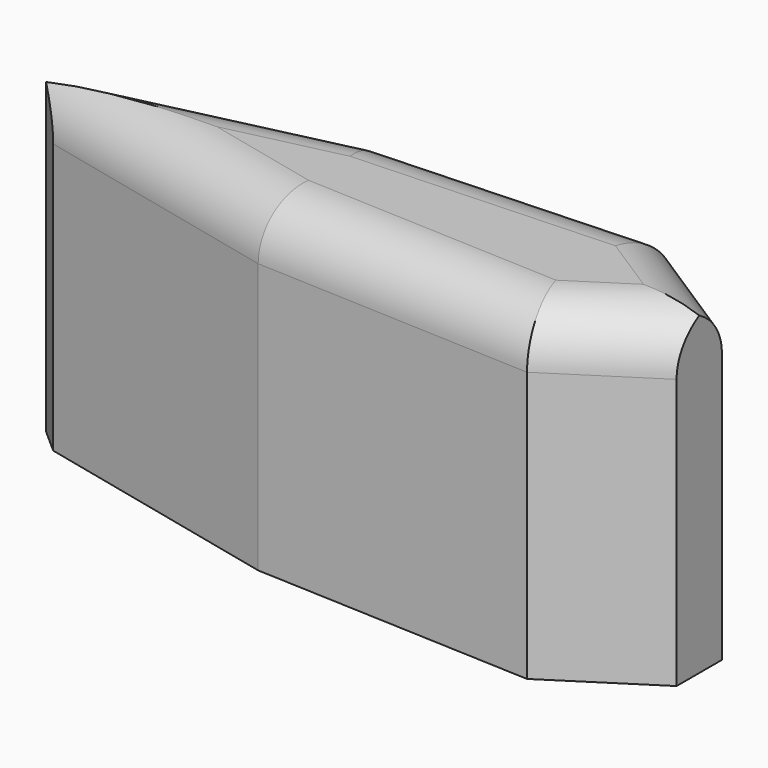
from build123d import *

# Parameters (mm, degrees)
F1_DEPTH     = 30
F2_T1_DEPTH  = 75.8181276712
F2_T3_DEPTH  = 75.8181276712
F2_T5_DEPTH  = 73.9035501151
F2_T7_DEPTH  = 35.8710514752
F2_T9_DEPTH  = 73.9035501151
F2_T11_DEPTH = 35.8710514752


# Not quite as in the source:
# - a fillet or chamfer that OpenCascade refuses, or shapes differently, is made with other operations: its cross-section is extruded or revolved along the edge and cut away or added


with BuildPart() as f1:
    # F0 (on Top) → F1 (new body)
    with BuildSketch(Plane.XY):
        Polygon((26.1299721897, 2.6230975054), (16.9895477593, 8.5080275312), (-8.8039748371, 7.3811253533), (-32.0932716131, 1.9970410503), (-34.347075969, 0), (-32.0932716131, -1.9970410503), (-8.8039748371, -7.3811253533), (16.9895477593, -8.5080275312), (26.1299721897, -2.6230975054), (26.1299721897, 0), align=None)
    extrude(amount=F1_DEPTH)

    # F2: fillet of radius 5 on 9 edges, made by hand

    # F2_s2 → F2_t1 (cut)
    with BuildSketch(Plane(origin=(-45.9296019103, 2.006634349, 0), x_dir=(0, 0, 1), z_dir=(0.9990469845, -0.0436477111, 0))):
        with BuildLine():
            ThreePointArc((30, 2.758364377), (28.5355339059, 6.2938982829), (25, 7.758364377))
            Line((25, 7.758364377), (30, 7.758364377))
            Line((30, 7.758364377), (30, 2.758364377))
        make_face()
    extrude(amount=F2_T1_DEPTH, mode=Mode.SUBTRACT)

    # F2_s4 → F2_t3 (cut)
    with BuildSketch(Plane(origin=(29.816269913, 1.3026533843, 0), x_dir=(0, 0, 1), z_dir=(-0.9990469845, -0.0436477111, 0))):
        with BuildLine():
            ThreePointArc((30, 2.758364377), (28.5355339059, 6.2938982829), (25, 7.758364377))
            Line((25, 7.758364377), (30, 7.758364377))
            Line((30, 7.758364377), (30, 2.758364377))
        make_face()
    extrude(amount=F2_T3_DEPTH, mode=Mode.SUBTRACT)

    # F2_s6 → F2_t5 (cut)
    with BuildSketch(Plane(origin=(-42.2055793243, 9.7572030329, 0), x_dir=(0, 0, 1), z_dir=(0.9743028405, -0.2252420363, 0))):
        with BuildLine():
            ThreePointArc((30, 4.174476618), (28.5355339059, 7.7100105239), (25, 9.174476618))
            Line((25, 9.174476618), (30, 9.174476618))
            Line((30, 9.174476618), (30, 4.174476618))
        make_face()
    extrude(amount=F2_T5_DEPTH, mode=Mode.SUBTRACT)

    # F2_s8 → F2_t7 (cut)
    with BuildSketch(Plane(origin=(27.7887436793, -17.8913805703, 0), x_dir=(0, 0, 1), z_dir=(-0.8408040796, 0.5413395419, 0))):
        with BuildLine():
            ThreePointArc((25, 16.3506982595), (28.5355339059, 14.8862321654), (30, 11.3506982595))
            Line((30, 11.3506982595), (30, 16.3506982595))
            Line((30, 16.3506982595), (25, 16.3506982595))
        make_face()
    extrude(amount=F2_T7_DEPTH, mode=Mode.SUBTRACT)

    # F2_s10 → F2_t9 (cut)
    with BuildSketch(Plane(origin=(29.7988594786, 6.8889830855, 0), x_dir=(0, 0, 1), z_dir=(-0.9743028405, -0.2252420363, 0))):
        with BuildLine():
            ThreePointArc((30, 4.174476618), (28.5355339059, 7.7100105239), (25, 9.174476618))
            Line((25, 9.174476618), (30, 9.174476618))
            Line((30, 9.174476618), (30, 4.174476618))
        make_face()
    extrude(amount=F2_T9_DEPTH, mode=Mode.SUBTRACT)

    # F2_s12 → F2_t11 (cut)
    with BuildSketch(Plane(origin=(-2.3717827422, -1.5270380036, 0), x_dir=(0, 0, 1), z_dir=(0.8408040796, 0.5413395419, 0))):
        with BuildLine():
            ThreePointArc((30, 11.3506982595), (28.5355339059, 14.8862321654), (25, 16.3506982595))
            Line((25, 16.3506982595), (30, 16.3506982595))
            Line((30, 16.3506982595), (30, 11.3506982595))
        make_face()
    extrude(amount=F2_T11_DEPTH, mode=Mode.SUBTRACT)


solid = f1.part
